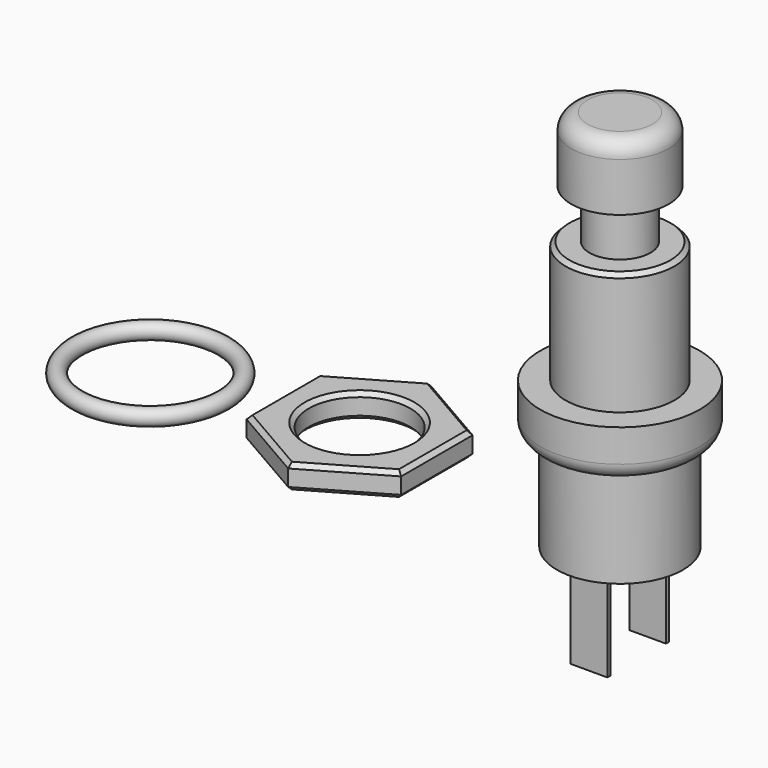
from build123d import *

# Parameters (mm, degrees)
F0_R      = 3.875
F0_R_2    = 3.35
F0_R_3    = 3
F0_W      = 2.25
F0_H      = 0.25
F0_R_4    = 1.875
F1_DEPTH  = 6.5
F2_START  = 6
F0_R_5    = 4.9
F2_DEPTH  = 3
F3_START  = 6
F3_DEPTH  = 10.5
F4_START  = 16.5
F4_DEPTH  = 7
F5_START  = 19.5
F5_DEPTH  = 4
F6_R      = 1
F7_R      = 1
F8_SIZE   = 0.25
F9_DEPTH  = 5.75
F10_R     = 3.125
F11_DEPTH = 1.5
F12_SIZE  = 0.25
F13_R     = 0.5


with BuildPart() as f1:
    # F0 (on Top) → F1 (new body)
    with BuildSketch(Plane.XY):
        Circle(F0_R)
        Circle(F0_R_2, mode=Mode.SUBTRACT)
        Circle(F0_R_2)
        Circle(F0_R_3, mode=Mode.SUBTRACT)
        Circle(F0_R_3)
        with Locations((0, -2.25)):
            Rectangle(F0_W, F0_H, mode=Mode.SUBTRACT)
        Circle(F0_R_4, mode=Mode.SUBTRACT)
        with Locations((0, 2.25)):
            Rectangle(F0_W, F0_H, mode=Mode.SUBTRACT)
        Circle(F0_R_4)
        with Locations((0, 2.25)):
            Rectangle(F0_W, F0_H)
        with Locations((0, -2.25)):
            Rectangle(F0_W, F0_H)
    extrude(amount=F1_DEPTH)

    # F0 (on Top) → F9 (join)
    with BuildSketch(Plane.XY):
        with Locations((0, 2.25)):
            Rectangle(F0_W, F0_H)
        with Locations((0, -2.25)):
            Rectangle(F0_W, F0_H)
    extrude(amount=-F9_DEPTH)


with BuildPart() as f2:
    # F0 (on Top) → F2 (new body)
    with BuildSketch(Plane.XY.offset(F2_START)):
        Circle(F0_R_5)
        Circle(F0_R, mode=Mode.SUBTRACT)
        Circle(F0_R)
        Circle(F0_R_2, mode=Mode.SUBTRACT)
        Circle(F0_R_2)
        Circle(F0_R_3, mode=Mode.SUBTRACT)
        Circle(F0_R_3)
        with Locations((0, -2.25)):
            Rectangle(F0_W, F0_H, mode=Mode.SUBTRACT)
        Circle(F0_R_4, mode=Mode.SUBTRACT)
        with Locations((0, 2.25)):
            Rectangle(F0_W, F0_H, mode=Mode.SUBTRACT)
        Circle(F0_R_4)
    extrude(amount=F2_DEPTH)

    # F0 (on Top) → F3 (join)
    with BuildSketch(Plane.XY.offset(F3_START)):
        Circle(F0_R_2)
        Circle(F0_R_3, mode=Mode.SUBTRACT)
        Circle(F0_R_3)
        with Locations((0, -2.25)):
            Rectangle(F0_W, F0_H, mode=Mode.SUBTRACT)
        Circle(F0_R_4, mode=Mode.SUBTRACT)
        with Locations((0, 2.25)):
            Rectangle(F0_W, F0_H, mode=Mode.SUBTRACT)
        with Locations((0, 2.25)):
            Rectangle(F0_W, F0_H)
        with Locations((0, -2.25)):
            Rectangle(F0_W, F0_H)
    extrude(amount=F3_DEPTH)

    # F7
    f7_edges = [f2.edges().sort_by_distance(p)[0] for p in [
        (-4.9, 0, 6),
    ]]
    fillet(f7_edges, radius=F7_R)

    # F8
    f8_edges = [f2.edges().sort_by_distance(p)[0] for p in [
        (-3.35, 0, 16.5),
    ]]
    chamfer(f8_edges, length=F8_SIZE)


with BuildPart() as f4:
    # F0 (on Top) → F4 (new body)
    with BuildSketch(Plane.XY.offset(F4_START)):
        Circle(F0_R_4)
    extrude(amount=F4_DEPTH)

    # F0 (on Top) → F5 (join)
    with BuildSketch(Plane.XY.offset(F5_START)):
        Circle(F0_R_3)
        with Locations((0, -2.25)):
            Rectangle(F0_W, F0_H, mode=Mode.SUBTRACT)
        Circle(F0_R_4, mode=Mode.SUBTRACT)
        with Locations((0, 2.25)):
            Rectangle(F0_W, F0_H, mode=Mode.SUBTRACT)
        Circle(F0_R_4)
        with Locations((0, -2.25)):
            Rectangle(F0_W, F0_H)
        with Locations((0, 2.25)):
            Rectangle(F0_W, F0_H)
    extrude(amount=F5_DEPTH)

    # F6
    f6_edges = [f4.edges().sort_by_distance(p)[0] for p in [
        (-3, 0, 23.5),
    ]]
    fillet(f6_edges, radius=F6_R)


with BuildPart() as f11:
    # F10 (on Top) → F11 (new body)
    with BuildSketch(Plane.XY):
        Polygon((-20.75, 2.7424137787), (-20.75, -2.7424137787), (-16, -5.4848275573), (-11.25, -2.7424137787), (-11.25, 2.7424137787), (-16, 5.4848275573), align=None)
        with Locations((-16, 0)):
            Circle(F10_R, mode=Mode.SUBTRACT)
    extrude(amount=F11_DEPTH)

    # F12
    f12_edges = [f11.edges().sort_by_distance(p)[0] for p in [
        (-20.75, 0, 1.5),
        (-18.375, -4.113621, 1.5),
        (-13.625, -4.113621, 1.5),
        (-11.25, 0, 1.5),
        (-13.625, 4.113621, 1.5),
        (-18.375, 4.113621, 1.5),
        (-19.125, 0, 1.5),
        (-20.75, 0, 0),
        (-18.375, -4.113621, 0),
        (-13.625, -4.113621, 0),
        (-11.25, 0, 0),
        (-13.625, 4.113621, 0),
        (-18.375, 4.113621, 0),
        (-19.125, 0, 0),
    ]]
    chamfer(f12_edges, length=F12_SIZE)


with BuildPart() as f15:
    # F13 (on Front) → F15 (revolve)
    with BuildSketch(Plane.XZ):
        with Locations((-24.3600804166, 0)):
            Circle(F13_R)
    revolve(axis=Axis((-28.8600804166, 0, 0), (0, 0, 1)))


solid = Compound([f1.part, f2.part, f4.part, f11.part, f15.part])
